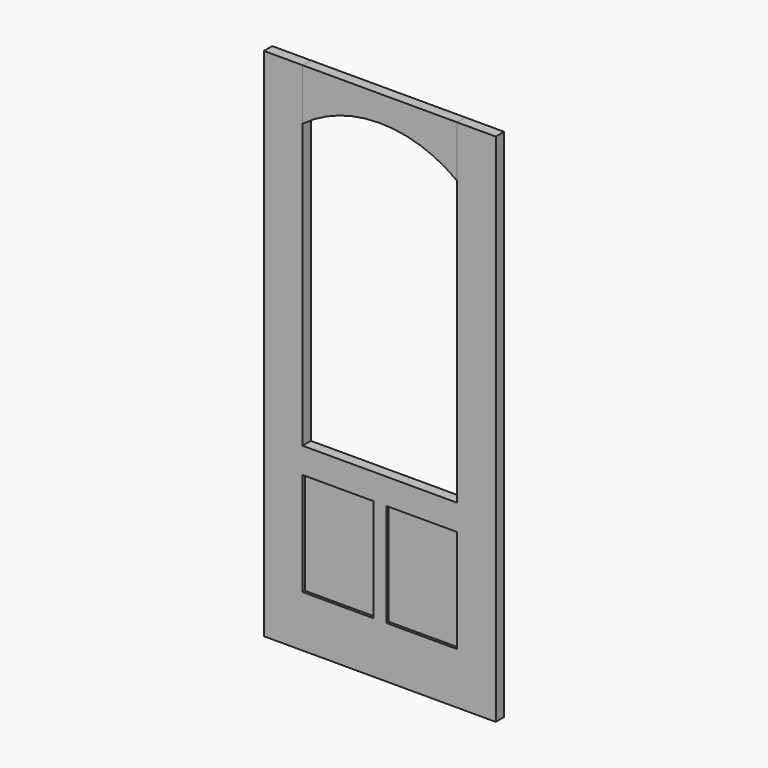
from build123d import *

# Parameters (mm, degrees)
F1_DEPTH = 41.275
F4_DEPTH = 41.275
F5_W     = 279.4
F5_H     = 406.4
F6_DEPTH = 41.276
F7_W     = 279.4
F7_H     = 406.4
F8_DEPTH = 9.525


# Not quite as in the source:
# - a length typed as a fraction of an inch, garbled in the dataset ("3 / 203.2 mm" for 3/8 in), is restored


with BuildPart() as f1:
    # F0 (on Front) → F1 (new body)
    with BuildSketch(Plane.XZ):
        Polygon((0, 2032), (0, 0), (914.4, 0), (914.4, 2032), (762, 2032), (762, 711.2), (152.4, 711.2), (152.4, 2032), align=None)
    extrude(amount=F1_DEPTH)

    # F5 (on Front) → F6 (cut, through all)
    with BuildSketch(Plane.XZ):
        with Locations((622.3, 406.4)):
            Rectangle(F5_W, F5_H)
        with Locations((292.1, 406.4)):
            Rectangle(F5_W, F5_H)
    extrude(amount=F6_DEPTH, mode=Mode.SUBTRACT)


with BuildPart() as f4:
    # F3 (on Front) → F4 (new body, through all)
    with BuildSketch(Plane.XZ):
        with BuildLine():
            Line((762, 2032), (152.4, 2032))
            Line((152.4, 2032), (152.4, 1828.8))
            ThreePointArc((152.4, 1828.8), (457.2, 1930.4), (762, 1828.8))
            Line((762, 1828.8), (762, 2032))
        make_face()
    extrude(amount=F4_DEPTH)


with BuildPart() as f8:
    # F7 (on offset) → F8 (new body, symmetric)
    with BuildSketch(Plane.XZ.offset(20.6375)):
        with Locations((292.1, 406.4)):
            Rectangle(F7_W, F7_H)
    extrude(amount=F8_DEPTH, both=True)


with BuildPart() as f8b:
    # F7 (on offset) → F8, piece 2 (new body, symmetric)
    with BuildSketch(Plane.XZ.offset(20.6375)):
        with Locations((622.3, 406.4)):
            Rectangle(F7_W, F7_H)
    extrude(amount=F8_DEPTH, both=True)


solid = Compound([f1.part, f4.part, f8.part, f8b.part])
